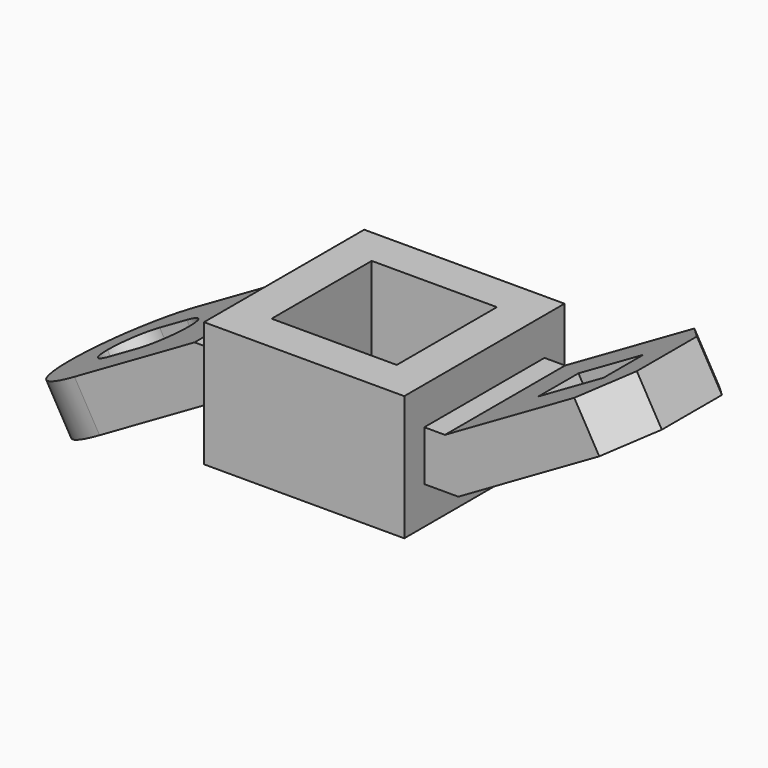
from build123d import *

# Parameters (mm, degrees)
F0_W      = 50.8
F0_H      = 50.8
F0_W_2    = 31.75
F0_H_2    = 31.75
F1_DEPTH  = 15.875
F3_DEPTH  = 19.05
F5_DEPTH  = 25.4
F6_R      = 19.04999
F7_W      = 19.05
F7_H      = 12.7
F8_DEPTH  = 56.6950905122
F9_SIZE   = 9.525
F10_DEPTH = 38.101


# Not quite as in the source:
# - a fillet or chamfer is up to 0.001 mm smaller than in the source, because OpenCascade refuses the exact size


with BuildPart() as f1:
    # F0 (on Top) → F1 (new body, symmetric)
    with BuildSketch(Plane.XY):
        Rectangle(F0_W, F0_H)
        Rectangle(F0_W_2, F0_H_2, mode=Mode.SUBTRACT)
    extrude(amount=F1_DEPTH, both=True)

    # F2 (on Front) → F3 (join, symmetric)
    with BuildSketch(Plane.XZ):
        Polygon((-73.4620968847, -31.75), (-29.4680063725, -6.35), (34.0319936275, -6.35), (78.0260841398, 19.05), (71.6760841398, 30.0485226281), (30.6290388837, 6.35), (-32.8709611163, 6.35), (-79.8120968847, -20.7514773719), align=None)
    extrude(amount=F3_DEPTH, both=True)

    # F4 (on face) → F5 (cut)
    with BuildSketch(Plane(origin=(-10.9673709361, 0, 18.9960436868), x_dir=(0.8660254038, 0, 0.5), z_dir=(-0.5, 0, 0.8660254038))):
        with BuildLine():
            Line((-52.5075421174, 7.9375), (-60.4450421174, 7.9375))
            ThreePointArc((-60.4450421174, 7.9375), (-66.0577021931, 5.6126600757), (-68.3825421174, 0))
            ThreePointArc((-68.3825421174, 0), (-66.0577021931, -5.6126600757), (-60.4450421174, -7.9375))
            Line((-60.4450421174, -7.9375), (-52.5075421174, -7.9375))
            ThreePointArc((-52.5075421174, -7.9375), (-44.5700421174, 0), (-52.5075421174, 7.9375))
        make_face()
    extrude(amount=-F5_DEPTH, mode=Mode.SUBTRACT)

    # F6 (radius 19.05 in the source; OpenCascade refuses exactly that, so slightly less here)
    f6_edges = [f1.edges().sort_by_distance(p)[0] for p in [
        (-76.637097, -19.05, -26.250739),
        (-76.637097, 19.05, -26.250739),
    ]]
    fillet(f6_edges, radius=F6_R)

    # F7 (on face) → F8 (cut, through all)
    with BuildSketch(Plane(origin=(4.9076290639, 0, -8.5002628834), x_dir=(0.8660254038, 0, 0.5), z_dir=(-0.5, 0, 0.8660254038))):
        with Locations((54.8725710229, 0)):
            Rectangle(F7_W, F7_H)
    extrude(amount=-F8_DEPTH, mode=Mode.SUBTRACT)

    # F9
    f9_edges = [f1.edges().sort_by_distance(p)[0] for p in [
        (74.851084, 19.05, 24.549261),
        (74.851084, -19.05, 24.549261),
    ]]
    chamfer(f9_edges, length=F9_SIZE)

    # F10 (cut, through all): a face of the model
    f10_faces = [f1.faces().sort_by_distance(p)[0] for p in [
        (0, 0, 6.35),
    ]]
    extrude(f10_faces, amount=-F10_DEPTH, mode=Mode.SUBTRACT)


solid = f1.part
